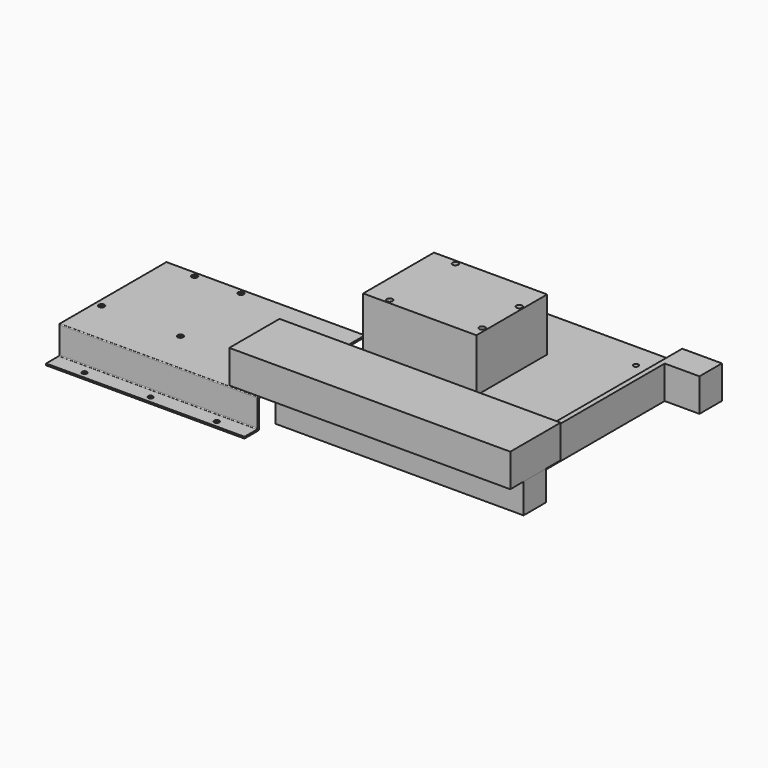
from build123d import *

# Parameters (mm, degrees)
F1_DEPTH  = 20
F2_R      = 1.5
F3_DEPTH  = 25
F6_DEPTH  = 120
F7_R      = 0.5
F8_R      = 1.5
F9_DEPTH  = 25
F10_W     = 125.9867332876
F10_H     = 8
F11_DEPTH = 166.4
F12_W     = 170
F12_H     = 38
F13_DEPTH = 20
F14_R     = 1.75
F15_DEPTH = 25
F16_R     = 2
F17_DEPTH = 5
F18_W     = 68.5
F18_H     = 53.5
F18_R     = 1.75
F19_DEPTH = 32
F20_ANGLE = -90


with BuildPart() as f1:
    # F0 (on Top) → F1 (new body)
    with BuildSketch(Plane.XY):
        Polygon((-75, -75), (75, -75), (75, -58), (54, -58), (54, 58), (75, 58), (75, 75), (-75, 75), align=None)
    extrude(amount=F1_DEPTH)

    # F2 (on face) → F3 (cut)
    with BuildSketch(Plane.XY.offset(20)):
        with Locations((-60, 60)):
            Circle(F2_R)
        with Locations((35, 60)):
            Circle(F2_R)
        with Locations((-60, -60)):
            Circle(F2_R)
        with Locations((35, -60)):
            Circle(F2_R)
    extrude(amount=-F3_DEPTH, mode=Mode.SUBTRACT)

    # F10 (on face) → F11 (cut)
    with BuildSketch(Plane.XZ.offset(75)):
        with Locations((-12.0066333562, 16)):
            Rectangle(F10_W, F10_H)
    extrude(amount=-F11_DEPTH, mode=Mode.SUBTRACT)


with BuildPart() as f6:
    # F5 (on offset) → F6 (new body)
    with BuildSketch(Plane(origin=(0, 35, 0), x_dir=(-1, 0, 0), z_dir=(0, 1, 0))):
        Polygon((78, 1), (78, 18), (-3, 18), (-3, 17), (77, 17), (77, 0), (88, 0), (88, 1), align=None)
    extrude(amount=-F6_DEPTH)

    # F7
    f7_edges = [f6.edges().sort_by_distance(p)[0] for p in [
        (-78, -25, 1),
        (-77, -25, 0),
        (-78, -25, 18),
        (-77, -25, 17),
    ]]
    fillet(f7_edges, radius=F7_R)

    # F8 (on face) → F9 (cut)
    with BuildSketch(Plane.XY.offset(1)):
        with Locations((-84, 15)):
            Circle(F8_R)
        with Locations((-84, -25)):
            Circle(F8_R)
        with Locations((-84, -65)):
            Circle(F8_R)
    extrude(amount=-F9_DEPTH, mode=Mode.SUBTRACT)

    # F14 (on face) → F15 (cut)
    with BuildSketch(Plane.XY.offset(18)):
        with Locations((-51, 31)):
            Circle(F14_R)
        with Locations((-52, -17.5)):
            Circle(F14_R)
        with Locations((0, -12.5)):
            Circle(F14_R)
        with Locations((0, 15.5)):
            Circle(F14_R)
    extrude(amount=-F15_DEPTH, mode=Mode.SUBTRACT)


with BuildPart() as f13:
    # F12 (on face) → F13 (new body)
    with BuildSketch(Plane.XY.offset(18)):
        with Locations((-10, -66)):
            Rectangle(F12_W, F12_H)
    extrude(amount=F13_DEPTH)

    # F16 (on face) → F17 (cut)
    with BuildSketch(Plane(origin=(-95, 0, 0), x_dir=(0, -1, 0), z_dir=(-1, 0, 0))):
        with Locations((58, 27)):
            Circle(F16_R)
    extrude(amount=-F17_DEPTH, mode=Mode.SUBTRACT)


with BuildPart() as f19:
    # F18 (on face) → F19 (new body)
    with BuildSketch(Plane.XY.offset(18)):
        with Locations((-31.75, 6.75)):
            Rectangle(F18_W, F18_H)
        with Locations((-52, -17.5)):
            Circle(F18_R, mode=Mode.SUBTRACT)
        with Locations((0, -12.5)):
            Circle(F18_R, mode=Mode.SUBTRACT)
        with Locations((-51, 31)):
            Circle(F18_R, mode=Mode.SUBTRACT)
        with Locations((0, 15.5)):
            Circle(F18_R, mode=Mode.SUBTRACT)
    extrude(amount=F19_DEPTH)


with BuildPart() as f6_1:
    # F20: moved
    add(f6.part.rotate(Axis((-77, -85, 8.5), (0, 0, -1)), F20_ANGLE))


solid = Compound([f1.part, f13.part, f19.part, f6_1.part])
